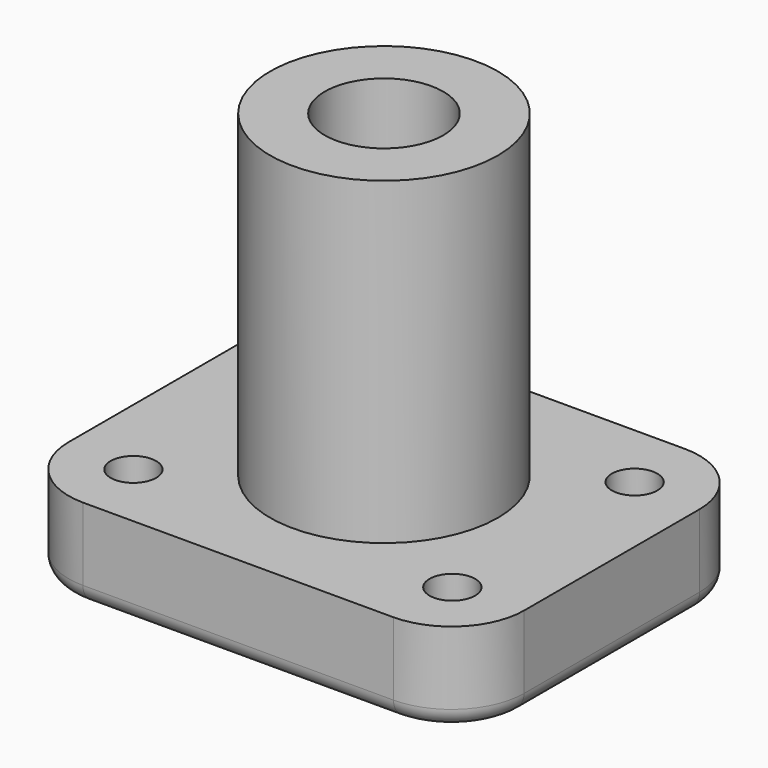
from build123d import *

# Parameters (mm, degrees)
F1_W           = 50
F1_H           = 40
F2_DEPTH       = 10
F3_T1_DEPTH    = 49.9995000031
F6_D           = 5
F6_DEPTH       = 20
F6_CSINK_D     = 10
F6_CSINK_ANGLE = 90
F6_TIP         = 1.5021515476
F7_R           = 2
F8_R           = 12.5
F8_R_2         = 6.5
F9_DEPTH       = 35
F10_DEPTH      = 25


# Not quite as in the source:
# - a fillet or chamfer that OpenCascade refuses, or shapes differently, is made with other operations: its cross-section is extruded or revolved along the edge and cut away or added


with BuildPart() as f2:
    # F1 (on Top) → F2 (new body)
    with BuildSketch(Plane.XY):
        Rectangle(F1_W, F1_H)
    extrude(amount=F2_DEPTH)

    # F3: fillet of radius 8 on 4 edges, made by hand

    # F3_s2 → F3_t1 (cut)
    with BuildSketch(Plane.XY.offset(-19.9997500016)):
        with BuildLine():
            ThreePointArc((-17.0001, 20.0001), (-22.6569542495, 17.6569542495), (-25.0001, 12.0001))
            Line((-25.0001, 12.0001), (-25.1601, 12.0001))
            ThreePointArc((-25.1601, 12.0001), (-25.16, 16.00005), (-25.16, 20))
            Line((-25.16, 20), (-25, 20.16))
            ThreePointArc((-25, 20.16), (-21.00005, 20.16), (-17.0001, 20.1601))
            Line((-17.0001, 20.1601), (-17.0001, 20.0001))
        make_face()
        with BuildLine():
            ThreePointArc((25.0001, 12.0001), (22.6569542495, 17.6569542495), (17.0001, 20.0001))
            Line((17.0001, 20.0001), (17.0001, 20.1601))
            ThreePointArc((17.0001, 20.1601), (21.00005, 20.16), (25, 20.16))
            Line((25, 20.16), (25.16, 20))
            ThreePointArc((25.16, 20), (25.16, 16.00005), (25.1601, 12.0001))
            Line((25.1601, 12.0001), (25.0001, 12.0001))
        make_face()
        with BuildLine():
            ThreePointArc((17.0001, -20.0001), (22.6569542495, -17.6569542495), (25.0001, -12.0001))
            Line((25.0001, -12.0001), (25.1601, -12.0001))
            ThreePointArc((25.1601, -12.0001), (25.16, -16.00005), (25.16, -20))
            Line((25.16, -20), (25, -20.16))
            ThreePointArc((25, -20.16), (21.00005, -20.16), (17.0001, -20.1601))
            Line((17.0001, -20.1601), (17.0001, -20.0001))
        make_face()
        with BuildLine():
            ThreePointArc((-17.0001, -20.0001), (-22.6569542495, -17.6569542495), (-25.0001, -12.0001))
            Line((-25.0001, -12.0001), (-25.1601, -12.0001))
            ThreePointArc((-25.1601, -12.0001), (-25.16, -16.00005), (-25.16, -20))
            Line((-25.16, -20), (-25, -20.16))
            ThreePointArc((-25, -20.16), (-21.00005, -20.16), (-17.0001, -20.1601))
            Line((-17.0001, -20.1601), (-17.0001, -20.0001))
        make_face()
    extrude(amount=F3_T1_DEPTH, mode=Mode.SUBTRACT)

    # F6
    with Locations(Plane(origin=(0, 0, 0), x_dir=(1, 0, 0), z_dir=(0, 0, -1))):
        with Locations((17.5, 12.5), (-17.5, 12.5), (-17.5, -12.5), (17.5, -12.5)):
            CounterSinkHole(F6_D / 2, F6_CSINK_D / 2, depth=F6_DEPTH, counter_sink_angle=F6_CSINK_ANGLE)
            with Locations((0, 0, -(F6_DEPTH + F6_TIP / 2))):  # 118° drill point
                Cone(0, F6_D / 2, F6_TIP, mode=Mode.SUBTRACT)

    # F7
    f7_edges = [f2.edges().sort_by_distance(p)[0] for p in [
        (0, -20, 0),
        (-22.656954, -17.656954, 0),
        (-25, 0, 0),
        (22.656954, -17.656954, 0),
        (-22.656954, 17.656954, 0),
        (25, 0, 0),
        (0, 20, 0),
        (22.656954, 17.656954, 0),
    ]]
    fillet(f7_edges, radius=F7_R)

    # F8 (on face) → F9 (join)
    with BuildSketch(Plane.XY.offset(10)):
        Circle(F8_R)
        Circle(F8_R_2, mode=Mode.SUBTRACT)
    extrude(amount=F9_DEPTH)

    # F10 (cut): a face of the model
    f10_faces = [f2.faces().sort_by_distance(p)[0] for p in [
        (0, 0, 10),
    ]]
    extrude(f10_faces, amount=-F10_DEPTH, mode=Mode.SUBTRACT)


solid = f2.part
